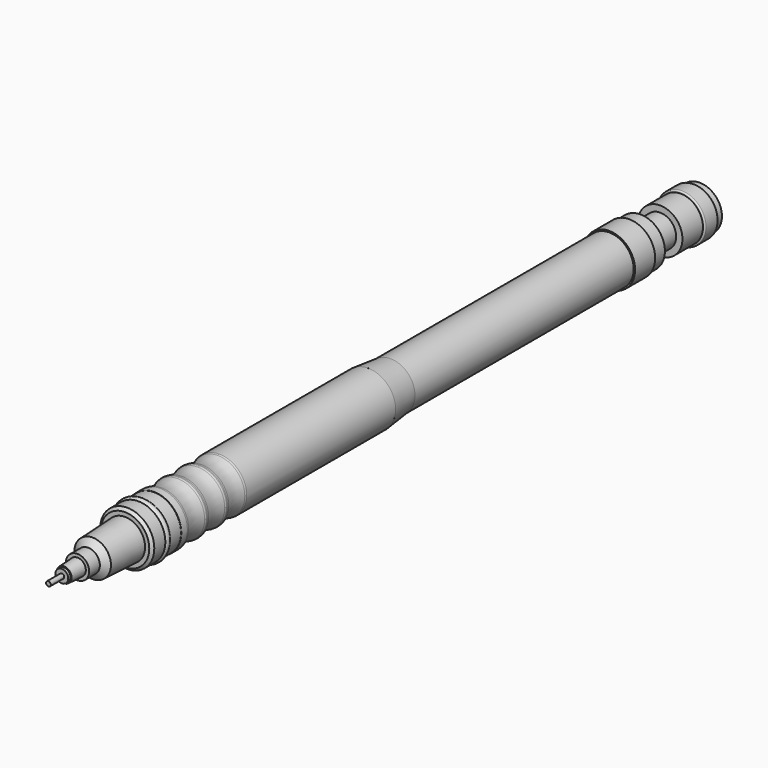
from build123d import *

# Parameters (mm, degrees)
F0_R      = 4.375
F1_DEPTH  = 56
F2_R      = 2.875
F3_DEPTH  = 4.4
F4_R      = 4
F5_DEPTH  = 4.6
F6_R      = 4.35
F7_DEPTH  = 3
F8_R      = 4
F9_DEPTH  = 1.25
F10_R     = 0.25
F11_R     = 4.375
F12_DEPTH = 5
F12_TAPER = -6
F13_R     = 4.9
F14_DEPTH = 48
F17_R     = 1
F18_R     = 4.85
F19_DEPTH = 6
F20_R     = 4.85
F21_DEPTH = 0.5
F21_TAPER = 45
F22_R     = 3.6
F23_DEPTH = 7.25
F23_TAPER = 2.5
F24_R     = 3.2835
F25_DEPTH = 1
F25_TAPER = 50
F26_R     = 2.0915
F27_DEPTH = 2.4
F28_R     = 1.5
F29_DEPTH = 3
F29_TAPER = 3
F30_R     = 1.15
F31_DEPTH = 0.5
F32_R     = 0.425
F33_DEPTH = 3
F35_R     = 4.625
F35_R_2   = 4.375
F36_DEPTH = 4.5
F37_R     = 0.625


with BuildPart() as f1:
    # F0 (on Front) → F1 (new body)
    with BuildSketch(Plane.XZ):
        Circle(F0_R)
    extrude(amount=F1_DEPTH)


with BuildPart() as f3:
    # F2 (on face) → F3 (new body)
    with BuildSketch(Plane(origin=(0, 0, 0), x_dir=(-1, 0, 0), z_dir=(0, 1, 0))):
        Circle(F2_R)
    extrude(amount=F3_DEPTH)


with BuildPart() as f5:
    # F4 (on face) → F5 (new body)
    with BuildSketch(Plane(origin=(0, 4.4, 0), x_dir=(-1, 0, 0), z_dir=(0, 1, 0))):
        Circle(F4_R)
    extrude(amount=F5_DEPTH)


with BuildPart() as f7:
    # F6 (on face) → F7 (new body)
    with BuildSketch(Plane(origin=(0, 9, 0), x_dir=(-1, 0, 0), z_dir=(0, 1, 0))):
        Circle(F6_R)
    extrude(amount=F7_DEPTH)

    # F10
    f10_edges = [f7.edges().sort_by_distance(p)[0] for p in [
        (4.35, 12, 0),
        (4.35, 9, 0),
    ]]
    fillet(f10_edges, radius=F10_R)


with BuildPart() as f9:
    # F8 (on face) → F9 (new body)
    with BuildSketch(Plane(origin=(0, 12, 0), x_dir=(-1, 0, 0), z_dir=(0, 1, 0))):
        Circle(F8_R)
    extrude(amount=F9_DEPTH)


with BuildPart() as f12:
    # F11 (on face) → F12 (new body)
    with BuildSketch(Plane.XZ.offset(56)):
        Circle(F11_R)
    extrude(amount=F12_DEPTH, taper=F12_TAPER)


with BuildPart() as f14:
    # F13 (on face) → F14 (new body)
    with BuildSketch(Plane.XZ.offset(61)):
        Circle(F13_R)
    extrude(amount=F14_DEPTH)

    # F15 (on Right) → F16 (revolve, cut)
    with BuildSketch(Plane.YZ):
        with BuildLine():
            ThreePointArc((-101, 11.6794494718), (-100.6266028276, 10.6180339887), (-100.5, 9.5))
            ThreePointArc((-100.5, 9.5), (-100.6266028276, 8.3819660113), (-101, 7.3205505282))
            ThreePointArc((-101, 7.3205505282), (-100.0632461982, 5.9923973242), (-98.75, 5.0348572251))
            ThreePointArc((-98.75, 5.0348572251), (-96.7426534085, 6.8779778796), (-96, 9.5))
            ThreePointArc((-96, 9.5), (-96.7426534085, 12.1220221204), (-98.75, 13.9651427749))
            ThreePointArc((-98.75, 13.9651427749), (-100.0632461982, 13.0076026758), (-101, 11.6794494718))
        make_face()
        with BuildLine():
            ThreePointArc((-101, 7.3205505282), (-101.5, 9.5), (-101, 11.6794494718))
            ThreePointArc((-101, 11.6794494718), (-101.9367538018, 13.0076026758), (-103.25, 13.9651427749))
            ThreePointArc((-103.25, 13.9651427749), (-106, 9.5), (-103.25, 5.0348572251))
            ThreePointArc((-103.25, 5.0348572251), (-101.9367538018, 5.9923973242), (-101, 7.3205505282))
        make_face()
        with BuildLine():
            ThreePointArc((-103.25, 13.9651427749), (-101.9367538018, 13.0076026758), (-101, 11.6794494718))
            ThreePointArc((-101, 11.6794494718), (-100.0632461982, 13.0076026758), (-98.75, 13.9651427749))
            ThreePointArc((-98.75, 13.9651427749), (-101, 14.5), (-103.25, 13.9651427749))
        make_face()
        with BuildLine():
            ThreePointArc((-98.75, 5.0348572251), (-100.0632461982, 5.9923973242), (-101, 7.3205505282))
            ThreePointArc((-101, 7.3205505282), (-101.9367538018, 5.9923973242), (-103.25, 5.0348572251))
            ThreePointArc((-103.25, 5.0348572251), (-101, 4.5), (-98.75, 5.0348572251))
        make_face()
        with BuildLine():
            ThreePointArc((-103.25, 5.0348572251), (-106, 9.5), (-103.25, 13.9651427749))
            ThreePointArc((-103.25, 13.9651427749), (-110.5, 9.5), (-103.25, 5.0348572251))
        make_face()
        with BuildLine():
            ThreePointArc((-91.5, 9.5), (-93.8779778796, 13.7573465915), (-98.75, 13.9651427749))
            ThreePointArc((-98.75, 13.9651427749), (-96.7426534085, 12.1220221204), (-96, 9.5))
            ThreePointArc((-96, 9.5), (-96.7426534085, 6.8779778796), (-98.75, 5.0348572251))
            ThreePointArc((-98.75, 5.0348572251), (-93.8779778796, 5.2426534085), (-91.5, 9.5))
        make_face()
    revolve(axis=Axis((0, -109, 0), (0, -1, 0)), mode=Mode.SUBTRACT)

    # F17
    f17_edges = [f14.edges().sort_by_distance(p)[0] for p in [
        (-3.464823, -103.540408, -3.464823),
        (3.464823, -103.540408, 3.464823),
        (3.464823, -107.459592, 3.464823),
        (-3.464823, -107.459592, -3.464823),
        (-3.464823, -94.540408, -3.464823),
        (3.464823, -94.540408, 3.464823),
        (3.464823, -98.459592, 3.464823),
        (-3.464823, -98.459592, -3.464823),
        (-3.464823, -99.040408, -3.464823),
        (3.464823, -99.040408, 3.464823),
        (3.464823, -102.959592, 3.464823),
        (-3.464823, -102.959592, -3.464823),
    ]]
    fillet(f17_edges, radius=F17_R)


with BuildPart() as f19:
    # F18 (on face) → F19 (new body)
    with BuildSketch(Plane.XZ.offset(109)):
        Circle(F18_R)
    extrude(amount=F19_DEPTH)

    # F20 (on face) → F21 (join)
    with BuildSketch(Plane.XZ.offset(115)):
        Circle(F20_R)
    extrude(amount=F21_DEPTH, taper=F21_TAPER)

    # F22 (on face) → F23 (join)
    with BuildSketch(Plane.XZ.offset(115.5)):
        Circle(F22_R)
    extrude(amount=F23_DEPTH, taper=F23_TAPER)

    # F24 (on face) → F25 (join)
    with BuildSketch(Plane.XZ.offset(122.75)):
        Circle(F24_R)
    extrude(amount=F25_DEPTH, taper=F25_TAPER)

    # F26 (on face) → F27 (join)
    with BuildSketch(Plane.XZ.offset(123.75)):
        Circle(F26_R)
    extrude(amount=F27_DEPTH)


with BuildPart() as f29:
    # F28 (on face) → F29 (new body)
    with BuildSketch(Plane.XZ.offset(126.15)):
        Circle(F28_R)
    extrude(amount=F29_DEPTH, taper=F29_TAPER)


with BuildPart() as f31:
    # F30 (on face) → F31 (new body)
    with BuildSketch(Plane.XZ.offset(129.15)):
        Circle(F30_R)
    extrude(amount=F31_DEPTH)

    # F32 (on face) → F33 (join)
    with BuildSketch(Plane.XZ.offset(129.65)):
        Circle(F32_R)
    extrude(amount=F33_DEPTH)


with BuildPart() as f36:
    # F35 (on offset) → F36 (new body)
    with BuildSketch(Plane.XZ.offset(2.5)):
        Circle(F35_R)
        Circle(F35_R_2, mode=Mode.SUBTRACT)
    extrude(amount=F36_DEPTH)


with BuildPart() as f38:
    # F37 (on Right) → F38 (revolve)
    with BuildSketch(Plane.YZ):
        with Locations((-112, 4.5)):
            Circle(F37_R)
    revolve(axis=Axis((0, -109, 0), (0, 1, 0)))


solid = Compound([f1.part, f3.part, f5.part, f7.part, f9.part, f12.part, f14.part, f19.part, f29.part, f31.part, f36.part, f38.part])
